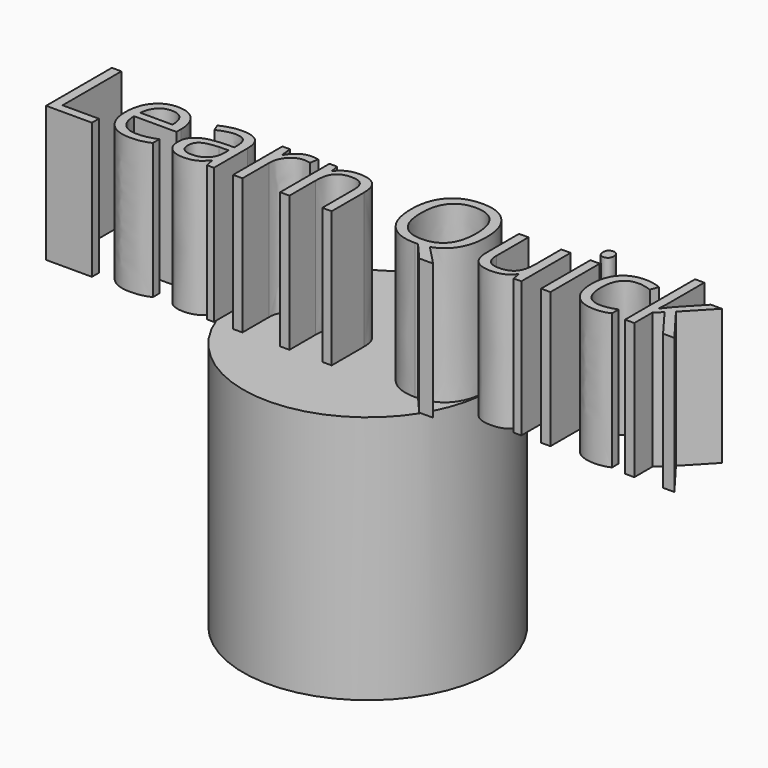
from build123d import *

# Parameters (mm, degrees)
F0_W         = 25.4
F0_H         = 50.8
F3_TEXT_SIZE = 23.4914756018
F4_DEPTH     = 27.686


# Not quite as in the source:
# - Text() gives the source's letters only with a copy of the font that has no kerning and outlines rounded to 1/6400 em; it was checked with that copy


with BuildPart() as f1:
    # F0 (on Front) → F1 (revolve)
    with BuildSketch(Plane.XZ):
        with Locations((12.7, 25.4)):
            Rectangle(F0_W, F0_H)
    revolve(axis=Axis((0, 0, 25.4), (0, 0, 1)))

    # F3 (on face) → F4 (join)
    with BuildSketch(Plane.XY.offset(50.8)):
        with Locations((-60.3731423616, -9.4309132546)):
            Text('Learn Quick', F3_TEXT_SIZE, font='Open Sans', text_align=(TextAlign.LEFT, TextAlign.BOTTOM))
    extrude(amount=F4_DEPTH)


solid = f1.part
